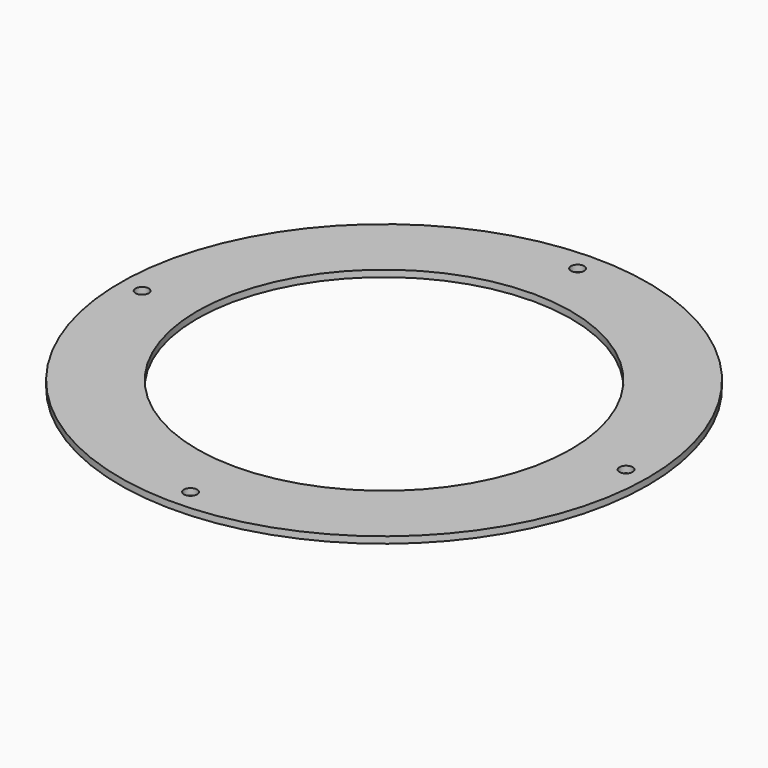
from build123d import *

# Parameters (mm, degrees)
F0_R     = 120
F0_R_2   = 3
F0_R_3   = 85
F1_DEPTH = 3


# Not quite as in the source:
# - a feature names something its author has since deleted; it is built from what else it names


with BuildPart() as f1:
    # F0 (on Top) → F1 (new body)
    with BuildSketch(Plane.XY):
        Circle(F0_R)
        with Locations((0, -110)):
            Circle(F0_R_2, mode=Mode.SUBTRACT)
        with Locations((-110, 0)):
            Circle(F0_R_2, mode=Mode.SUBTRACT)
        Circle(F0_R_3, mode=Mode.SUBTRACT)
        with Locations((110, 0)):
            Circle(F0_R_2, mode=Mode.SUBTRACT)
        with Locations((0, 110)):
            Circle(F0_R_2, mode=Mode.SUBTRACT)
    extrude(amount=F1_DEPTH)


solid = f1.part
